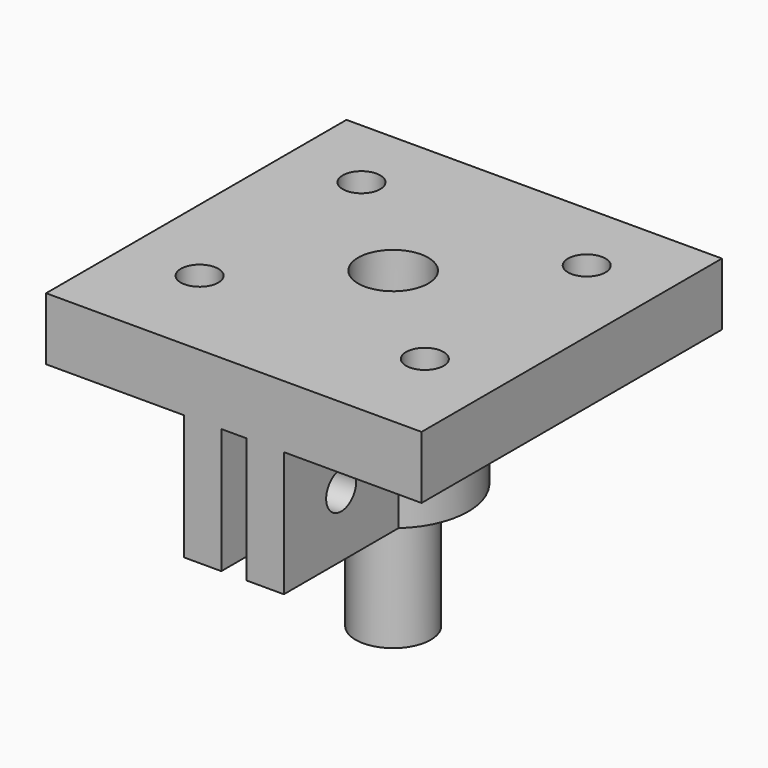
from build123d import *

# Parameters (mm, degrees)
F0_R     = 3
F0_R_2   = 2.8
F1_DEPTH = 20
F4_DEPTH = 10
F5_R     = 1.5
F6_DEPTH = 10.001
F7_W     = 30
F7_H     = 30
F7_R     = 1.5
F7_R_2   = 2.8
F8_DEPTH = 5


with BuildPart() as f1:
    # F0 (on Top) → F1 (new body)
    with BuildSketch(Plane.XY):
        Circle(F0_R)
        Circle(F0_R_2, mode=Mode.SUBTRACT)
    extrude(amount=F1_DEPTH)


with BuildPart() as f4:
    # F3 (on offset) → F4 (new body)
    with BuildSketch(Plane.XY.offset(10)):
        with BuildLine():
            ThreePointArc((-1, -2.8284271247), (-1.7320508076, 2.4494897428), (3, 0))
            ThreePointArc((3, 0), (2.4494897428, -1.7320508076), (1, -2.8284271247))
            Line((1, -2.8284271247), (1, -5.9160797831))
            Line((1, -5.9160797831), (1, -15.9160797831))
            Line((1, -15.9160797831), (4, -15.9160797831))
            Line((4, -15.9160797831), (4, -4.472135955))
            ThreePointArc((4, -4.472135955), (0, 6), (-4, -4.472135955))
            Line((-4, -4.472135955), (-4, -15.9160797831))
            Line((-4, -15.9160797831), (-1, -15.9160797831))
            Line((-1, -15.9160797831), (-1, -5.9160797831))
            Line((-1, -5.9160797831), (-1, -2.8284271247))
        make_face()
    extrude(amount=F4_DEPTH)

    # F5 (on face) → F6 (cut, through all)
    with BuildSketch(Plane.YZ.offset(4)):
        with Locations((-10.194107869, 15)):
            Circle(F5_R)
    extrude(amount=-F6_DEPTH, mode=Mode.SUBTRACT)

    # F7 (on face) → F8 (join)
    with BuildSketch(Plane.XY.offset(20)):
        with Locations((0, -0.9160797831)):
            Rectangle(F7_W, F7_H)
        with Locations((-9, -8.0839202169)):
            Circle(F7_R, mode=Mode.SUBTRACT)
        with Locations((9, -8.0839202169)):
            Circle(F7_R, mode=Mode.SUBTRACT)
        with Locations((-9, 8.0839202169)):
            Circle(F7_R, mode=Mode.SUBTRACT)
        Circle(F7_R_2, mode=Mode.SUBTRACT)
        with Locations((9, 8.0839202169)):
            Circle(F7_R, mode=Mode.SUBTRACT)
    extrude(amount=F8_DEPTH)


solid = Compound([f1.part, f4.part])
